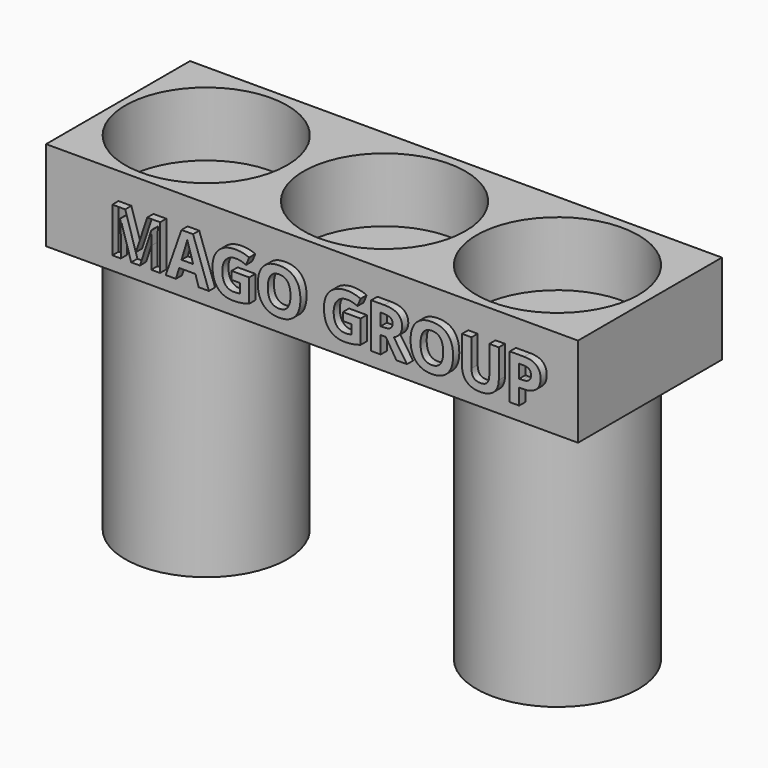
from build123d import *

# Parameters (mm, degrees)
F0_R         = 31.5
F1_DEPTH     = 10
F0_W         = 207
F0_H         = 70
F2_DEPTH     = 35
F3_TEXT_SIZE = 24.3573604772
F4_DEPTH     = 3
F5_DEPTH     = 100


# Not quite as in the source:
# - Text() gives the source's letters only with a copy of the font that has no kerning and outlines rounded to 1/6400 em; it was checked with that copy


with BuildPart() as f1:
    # F0 (on Top) → F1 (new body)
    with BuildSketch(Plane.XY):
        with Locations((-64.3688032488, 9.7374534234)):
            Circle(F0_R)
    extrude(amount=F1_DEPTH)


with BuildPart() as f1b:
    # F0 (on Top) → F1, piece 2 (new body)
    with BuildSketch(Plane.XY):
        with Locations((4.9999998882, 9.7374534234)):
            Circle(F0_R)
    extrude(amount=F1_DEPTH)


with BuildPart() as f1c:
    # F0 (on Top) → F1, piece 3 (new body)
    with BuildSketch(Plane.XY):
        with Locations((72.3037496209, 9.7374534234)):
            Circle(F0_R)
    extrude(amount=F1_DEPTH)


with BuildPart() as f2:
    # F0 (on Top) → F2 (new body)
    with BuildSketch(Plane.XY):
        with Locations((4.7417420745, 9.8165309429)):
            Rectangle(F0_W, F0_H)
        with Locations((-64.3688032488, 9.7374534234)):
            Circle(F0_R, mode=Mode.SUBTRACT)
        with Locations((4.9999998882, 9.7374534234)):
            Circle(F0_R, mode=Mode.SUBTRACT)
        with Locations((72.3037496209, 9.7374534234)):
            Circle(F0_R, mode=Mode.SUBTRACT)
    extrude(amount=F2_DEPTH)

    # F3 (on face) → F4 (join)
    with BuildSketch(Plane.XZ.offset(25.1834690571)):
        with Locations((-72.7701485157, 7.2746295482)):
            Text('MAGO GROUP', F3_TEXT_SIZE, font='Open Sans', font_style=FontStyle.BOLD, text_align=(TextAlign.LEFT, TextAlign.BOTTOM))
    extrude(amount=F4_DEPTH)


with BuildPart() as f5:
    # F5 (new): a face of the model
    f5_faces = [f1.part.faces().sort_by_distance(p)[0] for p in [
        (-64.3688032488, 9.7374534234, 0),
    ]]
    extrude(f5_faces, amount=F5_DEPTH)


with BuildPart() as f5b:
    # F5#2 (new): a face of the model
    f5_2_faces = [f1c.part.faces().sort_by_distance(p)[0] for p in [
        (72.3037496209, 9.7374534234, 0),
    ]]
    extrude(f5_2_faces, amount=F5_DEPTH)


solid = Compound([f1.part, f1b.part, f1c.part, f2.part, f5.part, f5b.part])
